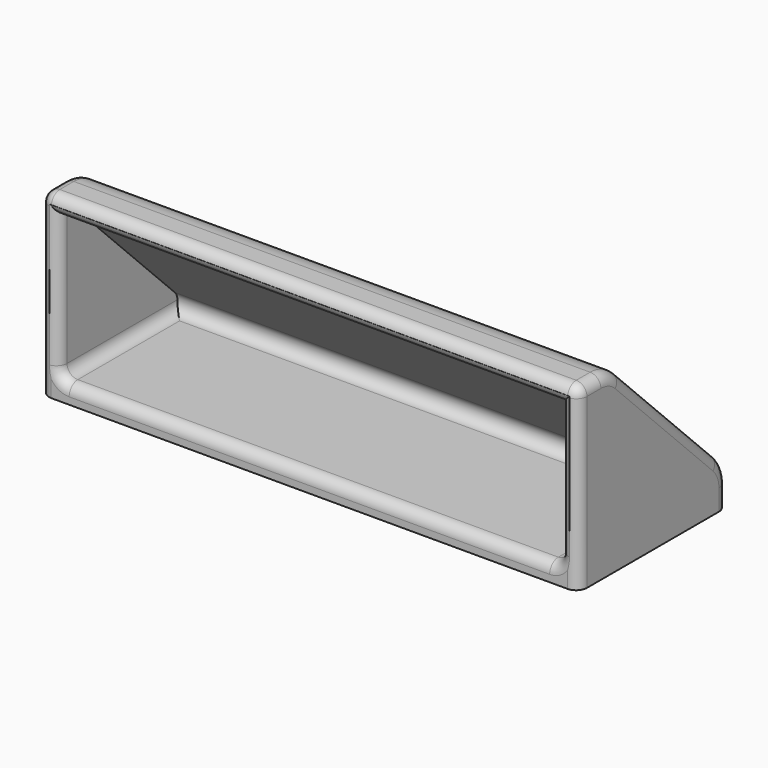
from build123d import *

# Parameters (mm, degrees)
F0_W         = 75
F0_H         = 26
F1_DEPTH     = 25
F2_SIZE      = 20
F3_W         = 70
F3_H         = 20
F4_DEPTH     = 23
F6_DEPTH     = 72.5
F7_T3_DEPTH  = 26.6167303864
F7_T7_DEPTH  = 26.6167303864
F7_T11_DEPTH = 79.0533008589
F7_T15_DEPTH = 73.1066017178
F7_S18_W     = 1.53
F7_S18_H     = 1.53
F7_T19_DEPTH = 1.53
F7_S23_W     = 1.53
F7_S23_H     = 1.53
F7_T24_DEPTH = 1.53
F7_T29_DEPTH = 27.25
F7_T32_DEPTH = 72
F7_T35_DEPTH = 67
F7_T38_DEPTH = 18.5
F7_T41_DEPTH = 18.5
F7_T44_DEPTH = 70
F7_T47_DEPTH = 27.25
F7_T50_DEPTH = 12.5
F7_T53_DEPTH = 35.7842712475
F7_T56_DEPTH = 8.25
F7_T59_DEPTH = 8.25
F7_T62_DEPTH = 35.7842712475
F7_T65_DEPTH = 12.5
F7_T68_ANGLE = 90
F7_T71_ANGLE = 90
F7_T75_DEPTH = 22.25
F7_T80_DEPTH = 73.75
F7_T87_DEPTH = 73.75
F7_T92_DEPTH = 22.25
F8_T1_DEPTH  = 75.0000000002
F8_T4_ANGLE  = 45
F8_T6_ANGLE  = 45
F8_T8_ANGLE  = 45
F8_T10_ANGLE = 45


# Not quite as in the source:
# - a fillet or chamfer that OpenCascade refuses, or shapes differently, is made with other operations: its cross-section is extruded or revolved along the edge and cut away or added
# - a feature names something its author has since deleted; it is built from what else it names


with BuildPart() as f1:
    # F0 (on Top) → F1 (new body)
    with BuildSketch(Plane.XY):
        Rectangle(F0_W, F0_H)
    extrude(amount=F1_DEPTH)

    # F2
    f2_edges = [f1.edges().sort_by_distance(p)[0] for p in [
        (0, 13, 25),
    ]]
    chamfer(f2_edges, length=F2_SIZE)

    # F3 (on face) → F4 (cut)
    with BuildSketch(Plane.XZ.offset(13)):
        with Locations((0, 12.4764153641)):
            Rectangle(F3_W, F3_H)
    extrude(amount=-F4_DEPTH, mode=Mode.SUBTRACT)

    # F5 (on face) → F6 (join)
    with BuildSketch(Plane(origin=(-37.5, 0, 0), x_dir=(0, -1, 0), z_dir=(-1, 0, 0))):
        Polygon((5.6137452684, 23.6137452684), (-10.4065692555, 7.5934307445), (-10.4065692555, 1.936576495), (7.2522564754, 19.5954022259), (11.2705995179, 23.6137452684), align=None)
    extrude(amount=-F6_DEPTH)

    # F7: fillet of radius 1.5 on 17 edges, made by hand


with BuildPart() as f7_tool1:
    # F7_s2 → F7_t3 (new body)
    with BuildSketch(Plane.XZ.offset(13)):
        with BuildLine():
            ThreePointArc((-35, 3.9764153641), (-34.5606601718, 2.9157551923), (-33.5, 2.4764153641))
            Line((-33.5, 2.4764153641), (-35, 2.4764153641))
            Line((-35, 2.4764153641), (-35, 3.9764153641))
        make_face()
    extrude(amount=-F7_T3_DEPTH)

    split(bisect_by=Plane.XZ.offset(-13), keep=Keep.TOP)


with BuildPart() as f7_tool5:
    # F7_s6 → F7_t7 (new body)
    with BuildSketch(Plane.XZ.offset(13)):
        with BuildLine():
            ThreePointArc((35, 3.9764153641), (34.5606601718, 2.9157551923), (33.5, 2.4764153641))
            Line((33.5, 2.4764153641), (35, 2.4764153641))
            Line((35, 2.4764153641), (35, 3.9764153641))
        make_face()
    extrude(amount=-F7_T7_DEPTH)

    split(bisect_by=Plane.XZ.offset(-13), keep=Keep.TOP)


with BuildPart() as f7_tool9:
    # F7_s10 → F7_t11 (new body)
    with BuildSketch(Plane.YZ.offset(35)):
        with BuildLine():
            ThreePointArc((7.3060702147, 5.0370755359), (7.6312293416, 3.4023902155), (6.2454100429, 2.4764153641))
            Line((6.2454100429, 2.4764153641), (9.8667303864, 2.4764153641))
            Line((9.8667303864, 2.4764153641), (7.3060702147, 5.0370755359))
        make_face()
    extrude(amount=-F7_T11_DEPTH)

    split(bisect_by=Plane.YZ.offset(-37.5), keep=Keep.TOP)


with BuildPart() as f7_tool13:
    # F7_s14 → F7_t15 (new body)
    with BuildSketch(Plane.YZ.offset(-36.5533008589)):
        with BuildLine():
            ThreePointArc((-9.6939297853, 22.0370755359), (-10.1805648086, 22.3622346628), (-10.7545899571, 22.4764153641))
            Line((-10.7545899571, 22.4764153641), (-10.1332696136, 22.4764153641))
            Line((-10.1332696136, 22.4764153641), (-9.6939297853, 22.0370755359))
        make_face()
    extrude(amount=F7_T15_DEPTH)


with BuildPart() as f1_1:
    add(f1.part)

    # F7_t16: union F7_tool1, F7_tool5, F7_tool9, F7_tool13
    add([f7_tool1.part, f7_tool5.part, f7_tool9.part, f7_tool13.part])


with BuildPart() as f7_tool17:
    # F7_s18 → F7_t19 (new body)
    with BuildSketch(Plane.YZ.offset(36)):
        with Locations((-12.265, 24.265)):
            Rectangle(F7_S18_W, F7_S18_H)
    extrude(amount=F7_T19_DEPTH)

    # F7_s20 → F7_t21 (revolve, cut)
    with BuildSketch(Plane(origin=(36, -11.5, 23.5), x_dir=(0, 0.7071067812, -0.7071067812), z_dir=(0, -0.7071067812, -0.7071067812))):
        with BuildLine():
            ThreePointArc((0, -1.5), (1.5, 0), (0, 1.5))
            Line((0, 1.5), (0, -1.5))
        make_face()
    revolve(axis=Axis((36, -11.5, 23.5), (1, 0, 0)), mode=Mode.SUBTRACT)


with BuildPart() as f7_tool22:
    # F7_s23 → F7_t24 (new body)
    with BuildSketch(Plane.XY.offset(23.5)):
        with Locations((-36.765, -12.265)):
            Rectangle(F7_S23_W, F7_S23_H)
    extrude(amount=F7_T24_DEPTH)

    # F7_s25 → F7_t26 (revolve, cut)
    with BuildSketch(Plane(origin=(-36, -11.5, 23.5), x_dir=(0.7071067812, 0.7071067812, 0), z_dir=(0.7071067812, -0.7071067812, 0))):
        with BuildLine():
            ThreePointArc((0, -1.5), (1.5, 0), (0, 1.5))
            Line((0, 1.5), (0, -1.5))
        make_face()
    revolve(axis=Axis((-36, -11.5, 23.5), (0, 0, 1)), mode=Mode.SUBTRACT)


with BuildPart() as f7_tool27:
    # F7_s28 → F7_t29 (new body)
    with BuildSketch(Plane.XY.offset(-3.75)):
        with BuildLine():
            ThreePointArc((37.5, -11.5), (37.0606601718, -12.5606601718), (36, -13))
            Line((36, -13), (37.5, -13))
            Line((37.5, -13), (37.5, -11.5))
        make_face()
    extrude(amount=F7_T29_DEPTH)


with BuildPart() as f7_tool30:
    # F7_s31 → F7_t32 (new body)
    with BuildSketch(Plane.YZ.offset(-36)):
        with BuildLine():
            ThreePointArc((-11.5, 25), (-12.5606601718, 24.5606601718), (-13, 23.5))
            Line((-13, 23.5), (-13, 25))
            Line((-13, 25), (-11.5, 25))
        make_face()
    extrude(amount=F7_T32_DEPTH)


with BuildPart() as f7_tool33:
    # F7_s34 → F7_t35 (new body)
    with BuildSketch(Plane.YZ.offset(-33.5)):
        with BuildLine():
            ThreePointArc((-13, 0.9764153641), (-12.5606601718, 2.0370755359), (-11.5, 2.4764153641))
            Line((-11.5, 2.4764153641), (-13, 2.4764153641))
            Line((-13, 2.4764153641), (-13, 0.9764153641))
        make_face()
    extrude(amount=F7_T35_DEPTH)


with BuildPart() as f7_tool36:
    # F7_s37 → F7_t38 (new body)
    with BuildSketch(Plane.XY.offset(3.9764153641)):
        with BuildLine():
            ThreePointArc((36.5, -13), (35.4393398282, -12.5606601718), (35, -11.5))
            Line((35, -11.5), (35, -13))
            Line((35, -13), (36.5, -13))
        make_face()
    extrude(amount=F7_T38_DEPTH)


with BuildPart() as f7_tool39:
    # F7_s40 → F7_t41 (new body)
    with BuildSketch(Plane.XY.offset(22.4764153641)):
        with BuildLine():
            ThreePointArc((-36.5, -13), (-35.4393398282, -12.5606601718), (-35, -11.5))
            Line((-35, -11.5), (-35, -13))
            Line((-35, -13), (-36.5, -13))
        make_face()
    extrude(amount=-F7_T41_DEPTH)


with BuildPart() as f7_tool42:
    # F7_s43 → F7_t44 (new body)
    with BuildSketch(Plane.YZ.offset(35)):
        with BuildLine():
            ThreePointArc((-13, 23.9764153641), (-12.5606601718, 22.9157551923), (-11.5, 22.4764153641))
            Line((-11.5, 22.4764153641), (-13, 22.4764153641))
            Line((-13, 22.4764153641), (-13, 23.9764153641))
        make_face()
    extrude(amount=-F7_T44_DEPTH)


with BuildPart() as f7_tool45:
    # F7_s46 → F7_t47 (new body)
    with BuildSketch(Plane.XY.offset(-3.75)):
        with BuildLine():
            ThreePointArc((-36, -13), (-37.0606601718, -12.5606601718), (-37.5, -11.5))
            Line((-37.5, -11.5), (-37.5, -13))
            Line((-37.5, -13), (-36, -13))
        make_face()
    extrude(amount=F7_T47_DEPTH)


with BuildPart() as f7_tool48:
    # F7_s49 → F7_t50 (new body)
    with BuildSketch(Plane.XY.offset(-3.75)):
        with BuildLine():
            ThreePointArc((37.5, 11.5), (37.0606601718, 12.5606601718), (36, 13))
            Line((36, 13), (37.5, 13))
            Line((37.5, 13), (37.5, 11.5))
        make_face()
    extrude(amount=F7_T50_DEPTH)


with BuildPart() as f7_tool51:
    # F7_s52 → F7_t53 (new body)
    with BuildSketch(Plane(origin=(0, 6.6516504294, -6.6516504294), x_dir=(1, 0, 0), z_dir=(0, -0.7071067812, 0.7071067812))):
        with BuildLine():
            ThreePointArc((37.5, 11.2279220614), (37.0606601718, 12.2885822331), (36, 12.7279220614))
            Line((36, 12.7279220614), (37.5, 12.7279220614))
            Line((37.5, 12.7279220614), (37.5, 11.2279220614))
        make_face()
    extrude(amount=F7_T53_DEPTH)


with BuildPart() as f7_tool54:
    # F7_s55 → F7_t56 (new body)
    with BuildSketch(Plane.XZ.offset(11.5)):
        with BuildLine():
            ThreePointArc((37.5, 23.5), (37.0606601718, 24.5606601718), (36, 25))
            Line((36, 25), (37.5, 25))
            Line((37.5, 25), (37.5, 23.5))
        make_face()
    extrude(amount=-F7_T56_DEPTH)


with BuildPart() as f7_tool57:
    # F7_s58 → F7_t59 (new body)
    with BuildSketch(Plane.XZ.offset(3.25)):
        with BuildLine():
            ThreePointArc((-36, 25), (-37.0606601718, 24.5606601718), (-37.5, 23.5))
            Line((-37.5, 23.5), (-37.5, 25))
            Line((-37.5, 25), (-36, 25))
        make_face()
    extrude(amount=F7_T59_DEPTH)


with BuildPart() as f7_tool60:
    # F7_s61 → F7_t62 (new body)
    with BuildSketch(Plane(origin=(0, 6.6516504294, -6.6516504294), x_dir=(1, 0, 0), z_dir=(0, -0.7071067812, 0.7071067812))):
        with BuildLine():
            ThreePointArc((-36, 12.7279220614), (-37.0606601718, 12.2885822331), (-37.5, 11.2279220614))
            Line((-37.5, 11.2279220614), (-37.5, 12.7279220614))
            Line((-37.5, 12.7279220614), (-36, 12.7279220614))
        make_face()
    extrude(amount=F7_T62_DEPTH)


with BuildPart() as f7_tool63:
    # F7_s64 → F7_t65 (new body)
    with BuildSketch(Plane.XY.offset(-3.75)):
        with BuildLine():
            ThreePointArc((-36, 13), (-37.0606601718, 12.5606601718), (-37.5, 11.5))
            Line((-37.5, 11.5), (-37.5, 13))
            Line((-37.5, 13), (-36, 13))
        make_face()
    extrude(amount=F7_T65_DEPTH)


with BuildPart() as f7_tool66:
    # F7_s67 → F7_t68 (revolve)
    with BuildSketch(Plane.XY.offset(3.9764153641)):
        with BuildLine():
            ThreePointArc((-36.5, -13), (-35.4393398282, -12.5606601718), (-35, -11.5))
            Line((-35, -11.5), (-35, -13))
            Line((-35, -13), (-36.5, -13))
        make_face()
    revolve(axis=Axis((-33.5, -13, 3.9764153641), (0, -1, 0)), revolution_arc=F7_T68_ANGLE)


with BuildPart() as f7_tool69:
    # F7_s70 → F7_t71 (revolve)
    with BuildSketch(Plane.XY.offset(3.9764153641)):
        with BuildLine():
            ThreePointArc((36.5, -13), (35.4393398282, -12.5606601718), (35, -11.5))
            Line((35, -11.5), (35, -13))
            Line((35, -13), (36.5, -13))
        make_face()
    revolve(axis=Axis((33.5, -13, 3.9764153641), (0, 1, 0)), revolution_arc=F7_T71_ANGLE)


with BuildPart() as f7_tool73:
    # F7_s74 → F7_t75 (new body)
    with BuildSketch(Plane.XY.offset(3.9764153641)):
        with BuildLine():
            ThreePointArc((36.5, -13), (35.4393398282, -12.5606601718), (35, -11.5))
            Line((35, -11.5), (35, -13))
            Line((35, -13), (36.5, -13))
        make_face()
    extrude(amount=F7_T75_DEPTH)

    split(bisect_by=Plane.XY.offset(25), keep=Keep.BOTTOM)

    split(bisect_by=Plane.XY.offset(22.4764153641), keep=Keep.TOP)


with BuildPart() as f7_tool78:
    # F7_s79 → F7_t80 (new body)
    with BuildSketch(Plane.YZ.offset(38.75)):
        with BuildLine():
            ThreePointArc((-13, 23.9764153641), (-12.5606601718, 22.9157551923), (-11.5, 22.4764153641))
            Line((-11.5, 22.4764153641), (-13, 22.4764153641))
            Line((-13, 22.4764153641), (-13, 23.9764153641))
        make_face()
    extrude(amount=-F7_T80_DEPTH)

    split(bisect_by=Plane.YZ.offset(37.5), keep=Keep.BOTTOM)

    split(bisect_by=Plane.YZ.offset(35), keep=Keep.TOP)


with BuildPart() as f7_tool73_1:
    add(f7_tool73.part)

    # F7_t83: intersect F7_tool78
    add(f7_tool78.part, mode=Mode.INTERSECT)


with BuildPart() as f7_tool85:
    # F7_s86 → F7_t87 (new body)
    with BuildSketch(Plane.YZ.offset(35)):
        with BuildLine():
            ThreePointArc((-13, 23.9764153641), (-12.5606601718, 22.9157551923), (-11.5, 22.4764153641))
            Line((-11.5, 22.4764153641), (-13, 22.4764153641))
            Line((-13, 22.4764153641), (-13, 23.9764153641))
        make_face()
    extrude(amount=-F7_T87_DEPTH)

    split(bisect_by=Plane.YZ.offset(-37.5), keep=Keep.TOP)

    split(bisect_by=Plane.YZ.offset(-35), keep=Keep.BOTTOM)


with BuildPart() as f7_tool90:
    # F7_s91 → F7_t92 (new body)
    with BuildSketch(Plane.XY.offset(26.2264153641)):
        with BuildLine():
            ThreePointArc((-36.5, -13), (-35.4393398282, -12.5606601718), (-35, -11.5))
            Line((-35, -11.5), (-35, -13))
            Line((-35, -13), (-36.5, -13))
        make_face()
    extrude(amount=-F7_T92_DEPTH)

    split(bisect_by=Plane.XY.offset(25), keep=Keep.BOTTOM)

    split(bisect_by=Plane.XY.offset(22.4764153641), keep=Keep.TOP)


with BuildPart() as f7_tool85_1:
    add(f7_tool85.part)

    # F7_t95: intersect F7_tool90
    add(f7_tool90.part, mode=Mode.INTERSECT)


with BuildPart() as f1_2:
    add(f1_1.part)

    # F7_t96: cut F7_tool17, F7_tool22, F7_tool27, F7_tool30, F7_tool33, F7_tool36, F7_tool39, F7_tool42, F7_tool45, F7_tool48, F7_tool51, F7_tool54, F7_tool57, F7_tool60, F7_tool63, F7_tool66, F7_tool69, F7_tool73, F7_tool85
    add([f7_tool17.part, f7_tool22.part, f7_tool27.part, f7_tool30.part, f7_tool33.part, f7_tool36.part, f7_tool39.part, f7_tool42.part, f7_tool45.part, f7_tool48.part, f7_tool51.part, f7_tool54.part, f7_tool57.part, f7_tool60.part, f7_tool63.part, f7_tool66.part, f7_tool69.part, f7_tool73_1.part, f7_tool85_1.part], mode=Mode.SUBTRACT)

    # F8: fillet of radius 5 on 2 edges, made by hand

    # F8_s2 → F8_t1 (cut)
    with BuildSketch(Plane.YZ.offset(-37.5000000001)):
        with BuildLine():
            ThreePointArc((13, 2.9289321881), (12.6193976626, 4.84234935), (11.5355339059, 6.4644660941))
            Line((11.5355339059, 6.4644660941), (13, 5))
            Line((13, 5), (13, 2.9289321881))
        make_face()
        with BuildLine():
            ThreePointArc((-5.5355339059, 23.5355339059), (-7.15765065, 24.6193976626), (-9.0710678119, 25))
            Line((-9.0710678119, 25), (-7, 25))
            Line((-7, 25), (-5.5355339059, 23.5355339059))
        make_face()
    extrude(amount=F8_T1_DEPTH, mode=Mode.SUBTRACT)

    # F8_s3 → F8_t4 (revolve, cut)
    with BuildSketch(Plane(origin=(0, -14.5355339059, 14.5355339059), x_dir=(1, 0, 0), z_dir=(0, 0.7071067812, -0.7071067812))):
        with BuildLine():
            ThreePointArc((37.5, -11.2279220614), (37.0606601718, -12.2885822332), (36.0000000001, -12.7279220614))
            Line((36.0000000001, -12.7279220614), (37.5, -12.7279220614))
            Line((37.5, -12.7279220614), (37.5, -11.2279220614))
        make_face()
    revolve(axis=Axis((37.5, -9.0710678119, 20), (1, 0, 0)), revolution_arc=F8_T4_ANGLE, mode=Mode.SUBTRACT)

    # F8_s5 → F8_t6 (revolve, cut)
    with BuildSketch(Plane.XZ.offset(9.0710678119)):
        with BuildLine():
            ThreePointArc((-37.5, 23.4999999999), (-37.0606601718, 24.5606601718), (-35.9999999999, 25))
            Line((-35.9999999999, 25), (-37.5, 25))
            Line((-37.5, 25), (-37.5, 23.4999999999))
        make_face()
    revolve(axis=Axis((-37.5, -9.0710678119, 20), (-1, 0, 0)), revolution_arc=F8_T6_ANGLE, mode=Mode.SUBTRACT)

    # F8_s7 → F8_t8 (revolve, cut)
    with BuildSketch(Plane.XY.offset(2.9289321881)):
        with BuildLine():
            ThreePointArc((37.5, 11.4999999999), (37.0606601718, 12.5606601718), (35.9999999999, 13))
            Line((35.9999999999, 13), (37.5, 13))
            Line((37.5, 13), (37.5, 11.4999999999))
        make_face()
    revolve(axis=Axis((37.5, 8, 2.9289321881), (1, 0, 0)), revolution_arc=F8_T8_ANGLE, mode=Mode.SUBTRACT)

    # F8_s9 → F8_t10 (revolve, cut)
    with BuildSketch(Plane(origin=(0, 2.5355339059, -2.5355339059), x_dir=(1, 0, 0), z_dir=(0, -0.7071067812, 0.7071067812))):
        with BuildLine():
            ThreePointArc((-37.5, 11.2279220613), (-37.0606601718, 12.2885822331), (-35.9999999999, 12.7279220614))
            Line((-35.9999999999, 12.7279220614), (-37.5, 12.7279220614))
            Line((-37.5, 12.7279220614), (-37.5, 11.2279220613))
        make_face()
    revolve(axis=Axis((-37.5, 8, 2.9289321881), (-1, 0, 0)), revolution_arc=F8_T10_ANGLE, mode=Mode.SUBTRACT)


solid = f1_2.part
